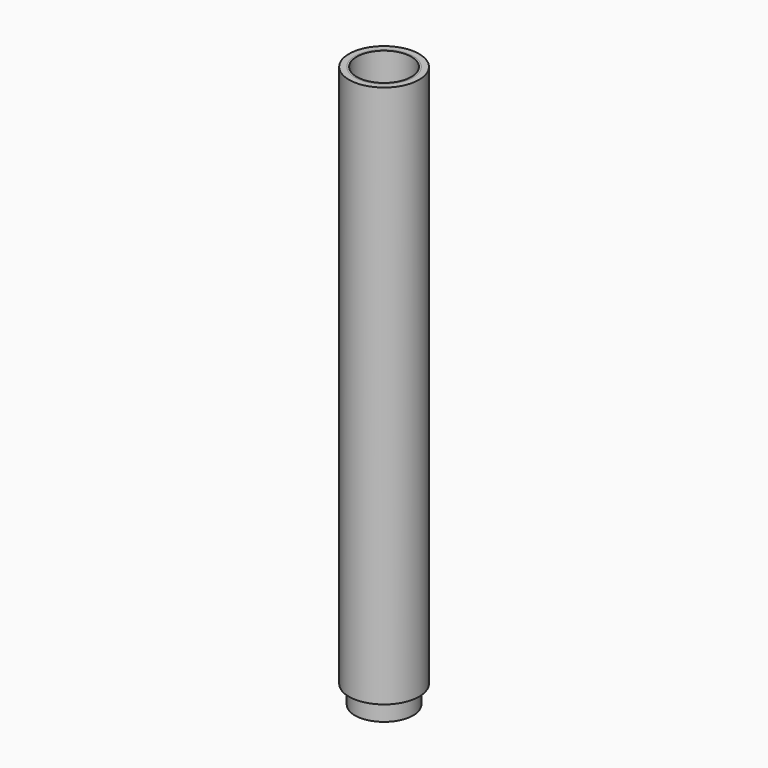
from build123d import *

# Parameters (mm, degrees)
F0_R     = 16.4061193369
F0_R_2   = 12.7740900069
F1_DEPTH = 254
F2_R     = 13.6249676804
F3_DEPTH = 262.636
F4_DEPTH = 61.722
F5_DEPTH = 50.292


with BuildPart() as f1:
    # F0 (on Top) → F1 (new body)
    with BuildSketch(Plane.XY):
        Circle(F0_R)
        Circle(F0_R_2, mode=Mode.SUBTRACT)
        Circle(F0_R_2)
    extrude(amount=-F1_DEPTH)

    # F0 (on Top) → F5 (cut)
    with BuildSketch(Plane.XY):
        Circle(F0_R_2)
    extrude(amount=-F5_DEPTH, mode=Mode.SUBTRACT)


with BuildPart() as f3:
    # F2 (on Top) → F3 (new body)
    with BuildSketch(Plane.XY):
        Circle(F2_R)
    extrude(amount=-F3_DEPTH)

    # F0 (on Top) → F4 (cut)
    with BuildSketch(Plane.XY):
        Circle(F0_R_2)
    extrude(amount=-F4_DEPTH, mode=Mode.SUBTRACT)


solid = Compound([f1.part, f3.part])
